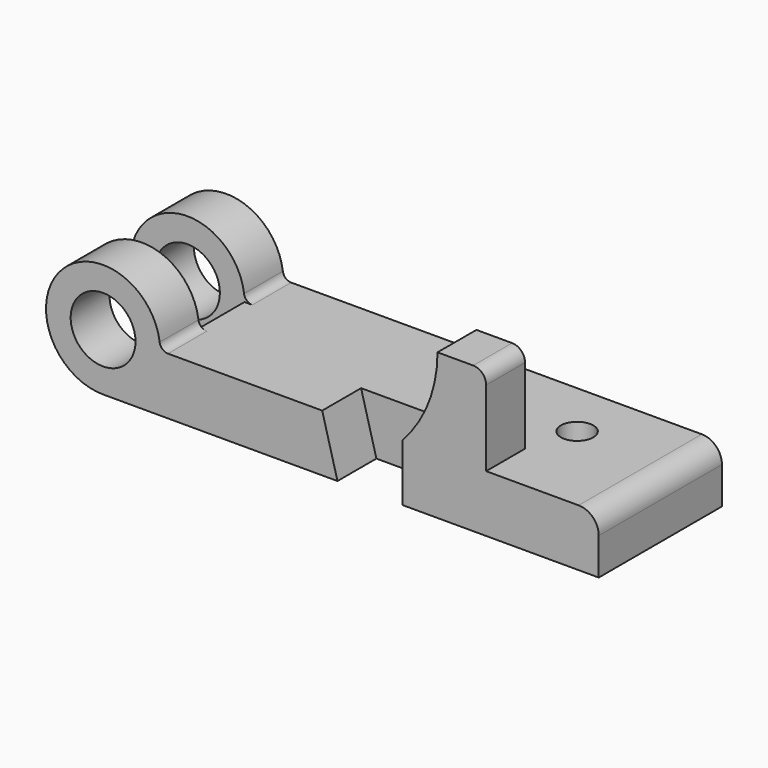
from build123d import *

# Parameters (mm, degrees)
F0_R     = 12.7
F1_DEPTH = 60.325
F2_W     = 32.8422
F2_H     = 41.275
F3_DEPTH = 34.798
F5_DEPTH = 19.05
F6_W     = 50.4518977821
F6_H     = 22.3266
F6_R     = 6.35
F7_DEPTH = 47.498
F8_R     = 3.302


with BuildPart() as f1:
    # F0 (on Front) → F1 (new body)
    with BuildSketch(Plane.XZ):
        with BuildLine():
            ThreePointArc((-79.7361564685, 22.352), (-117.8934072416, 38.1572507731), (-102.0881564685, 0))
            Line((-102.0881564685, 0), (92.1202435315, 0))
            Line((92.1202435315, 0), (92.1202435315, 14.478))
            ThreePointArc((92.1202435315, 14.478), (89.8140023266, 20.0457587951), (84.2462435315, 22.352))
            Line((84.2462435315, 22.352), (48.0004435315, 22.352))
            Line((48.0004435315, 22.352), (48.0004435315, 52.07))
            ThreePointArc((48.0004435315, 52.07), (46.5125459799, 55.6621024484), (42.9204435315, 57.15))
            Line((42.9204435315, 57.15), (28.9504435315, 57.15))
            ThreePointArc((28.9504435315, 57.15), (25.3762588931, 38.4343576341), (15.1582435315, 22.352))
            Line((15.1582435315, 22.352), (-79.7361564685, 22.352))
        make_face()
        with Locations((-102.0881564685, 22.352)):
            Circle(F0_R, mode=Mode.SUBTRACT)
    extrude(amount=-F1_DEPTH)

    # F2 (on face) → F3 (cut, through all)
    with BuildSketch(Plane.XY.offset(22.352)):
        with Locations((31.5793435315, 39.6875)):
            Rectangle(F2_W, F2_H)
    extrude(amount=F3_DEPTH, mode=Mode.SUBTRACT)

    # F4 (on Front) → F5 (cut)
    with BuildSketch(Plane.XZ):
        Polygon((15.1582435315, 0), (15.1582435315, 22.352), (-16.2361564685, 22.352), (-10.2417564685, 0), align=None)
    extrude(amount=-F5_DEPTH, mode=Mode.SUBTRACT)

    # F6 (on face) → F7 (cut, symmetric)
    with BuildSketch(Plane.XY.offset(22.352)):
        with Locations((-104.9621053595, 30.1625)):
            Rectangle(F6_W, F6_H)
        with Locations((53.2582435315, 37.973)):
            Circle(F6_R)
    extrude(amount=F7_DEPTH, both=True, mode=Mode.SUBTRACT)

    # F8
    f8_edges = [f1.edges().sort_by_distance(p)[0] for p in [
        (-79.736156, 9.4996, 22.352),
        (-79.736156, 50.8254, 22.352),
    ]]
    fillet(f8_edges, radius=F8_R)


solid = f1.part
